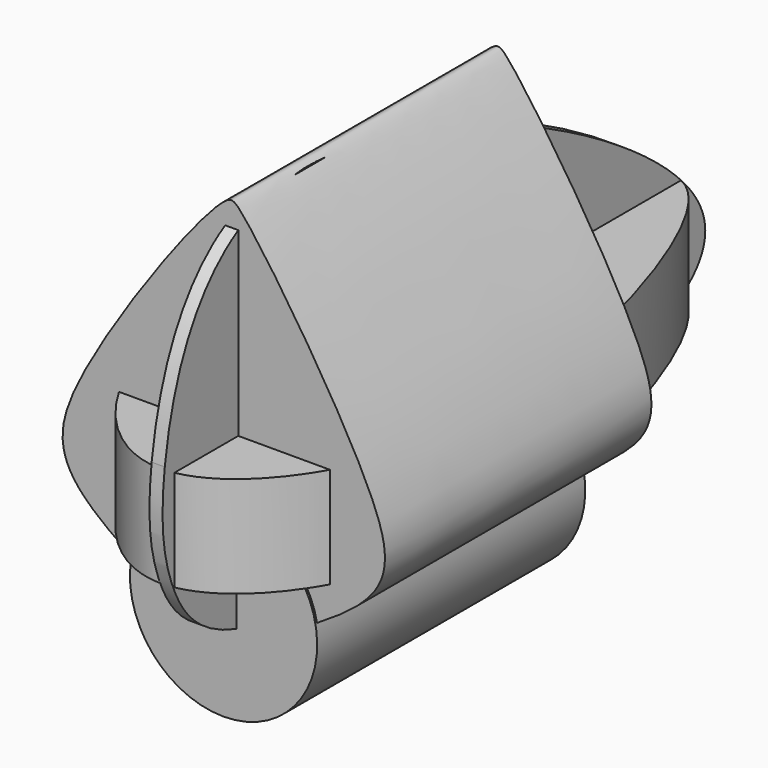
from build123d import *

# Parameters (mm, degrees)
F1_DEPTH = 25.4
F5_DEPTH = 3.302
F6_DEPTH = 83.82
F4_R     = 23.5632083166
F7_DEPTH = 84.328


# Not quite as in the source:
# - the program builds the solid bodies; features that only make, move or delete a surface that nothing else refers to are left out


with BuildPart() as f1:
    # F0 (on Top) → F1 (new body)
    with BuildSketch(Plane.XY):
        with BuildLine():
            Line((29.4822640717, -77.4155929685), (29.4822640717, 0))
            Line((29.4822640717, 0), (-29.1227447429, 0))
            add(Edge.make_bspline(
                [(-29.9289617687, -3.2632336952), (-29.667654713, -2.1806328695), (-29.3988189869, -1.0921885475), (-29.1227447429, 0)],
                knots=[0, 0, 0, 0, 0.0069135928, 0.0069135928, 0.0069135928, 0.0069135928], degree=3))
            Line((-29.9289617687, -3.2632336952), (-29.9289617687, -77.4155929685))
            Line((-29.9289617687, -77.4155929685), (29.4822640717, -77.4155929685))
        make_face()
        with BuildLine():
            add(Edge.make_bspline(
                [(29.4822640717, 0), (36.8093470661, -29.8029805077), (38.2405293985, -56.581996996), (29.4822640717, -77.4155929685)],
                knots=[0.3490618748, 0.3490618748, 0.3490618748, 0.3490618748, 0.5395897495, 0.5395897495, 0.5395897495, 0.5395897495], degree=3))
            Line((29.4822640717, 0), (29.4822640717, -77.4155929685))
        make_face()
        with BuildLine():
            Line((-29.1227447429, 0), (29.4822640717, 0))
            add(Edge.make_bspline(
                [(-29.1227447429, 0), (-22.3461187558, 26.8092857377), (0.1097970289, 85.4092558598), (22.8506074317, 26.9743271269), (29.4822640717, 0)],
                knots=[0.0069135928, 0.0069135928, 0.0069135928, 0.0069135928, 0.1766173363, 0.3490618748, 0.3490618748, 0.3490618748, 0.3490618748], degree=3))
        make_face()
        with BuildLine():
            add(Edge.make_bspline(
                [(-29.9289617687, -3.2632336952), (-29.667654713, -2.1806328695), (-29.3988189869, -1.0921885475), (-29.1227447429, 0)],
                knots=[0, 0, 0, 0, 0.0069135928, 0.0069135928, 0.0069135928, 0.0069135928], degree=3))
            Line((-29.1227447429, 0), (-29.9289617687, 0))
            Line((-29.9289617687, 0), (-29.9289617687, -3.2632336952))
        make_face()
        with BuildLine():
            add(Edge.make_bspline(
                [(29.4822640717, -77.4155929685), (23.1989903439, -92.3618387541), (0.0959929876, -116.1837405568), (-23.5848767505, -92.1405326762), (-29.9289617687, -77.4155929685)],
                knots=[0.5395897495, 0.5395897495, 0.5395897495, 0.5395897495, 0.6762764957, 0.8135309375, 0.8135309375, 0.8135309375, 0.8135309375], degree=3))
            Line((29.4822640717, -77.4155929685), (-29.9289617687, -77.4155929685))
        make_face()
        with BuildLine():
            Line((-29.9289617687, -77.4155929685), (-29.9289617687, -3.2632336952))
            add(Edge.make_bspline(
                [(-29.9289617687, -77.4155929685), (-38.5478127899, -57.410807208), (-36.9767707788, -32.462459996), (-29.9289617687, -3.2632336952)],
                knots=[0.8135309375, 0.8135309375, 0.8135309375, 0.8135309375, 1, 1, 1, 1], degree=3))
        make_face()
    extrude(amount=F1_DEPTH)

    # F2 (on Right) → F5 (join)
    with BuildSketch(Plane.YZ):
        with BuildLine():
            add(Edge.make_bspline(
                [(-106.9406792521, 27.9108993709), (-104.7699498582, 44.7842591168), (-85.999784023, 106.0820605098), (63.7740149004, 34.4520809419), (67.2044335068, -12.0750834044), (-82.9525104958, -30.0338929898), (-106.3787685917, -1.3125281144), (-108.4691524114, 16.029880231), (-106.9406792521, 27.9108993709)],
                knots=[0, 0, 0, 0, 0.1602136705, 0.4118548084, 0.5191699694, 0.7677684124, 0.8871889349, 1, 1, 1, 1], degree=3))
        make_face()
    extrude(amount=F5_DEPTH)

    # F3 (on Front) → F6 (join)
    with BuildSketch(Plane.XZ):
        with BuildLine():
            add(Edge.make_bspline(
                [(3.6589938682, -20.2464330941), (8.9055125534, -16.9597283327), (43.5124058761, -1.6812370703), (39.4368848502, 24.5814924516), (4.9136096926, 76.052816503), (-1.2031084613, 78.6514524427), (-40.3877816165, 25.2274980043), (-44.2918485042, -1.2674845253), (0.8590787196, -23.543526647), (1.9883011107, -21.2930459379), (3.6589938682, -20.2464330941)],
                knots=[0, 0, 0, 0, 0.1459804442, 0.2640492381, 0.4475385331, 0.4932619887, 0.6797496131, 0.8001112146, 0.9535142281, 1, 1, 1, 1], degree=3))
        make_face()
    extrude(amount=F6_DEPTH)

    # F4 (on Front) → F7 (join)
    with BuildSketch(Plane.XZ):
        with Locations((0, -14.0883298591)):
            Circle(F4_R)
    extrude(amount=F7_DEPTH)


solid = f1.part
